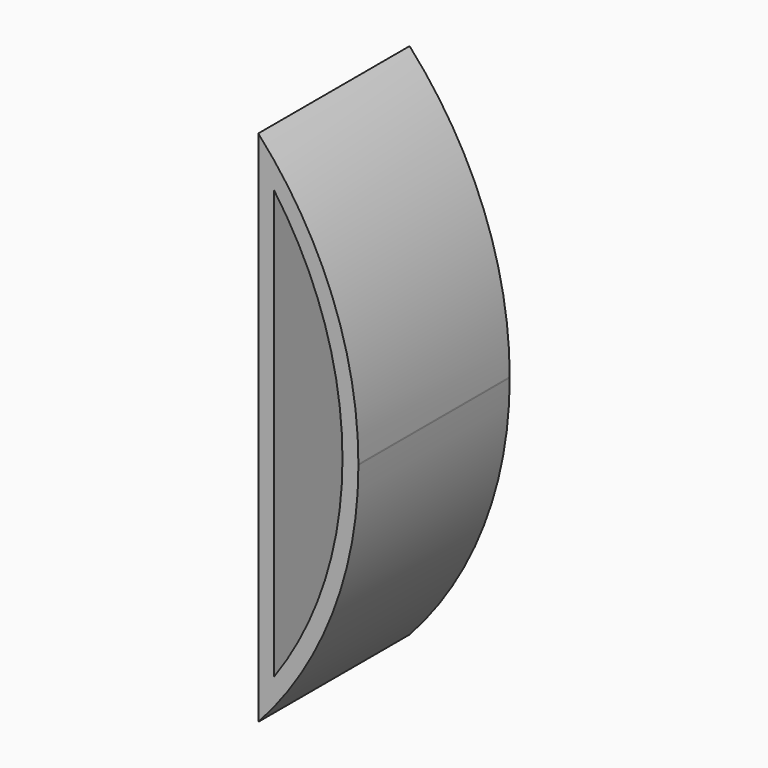
from build123d import *

# Parameters (mm, degrees)
F0_W        = 15.9461647272
F0_H        = 30.12368083
F1_DEPTH    = 82.5116038322
F2_T1_DEPTH = 236.0281493159
F3_T        = -2.54


# Not quite as in the source:
# - a fillet or chamfer that OpenCascade refuses, or shapes differently, is made with other operations: its cross-section is extruded or revolved along the edge and cut away or added


with BuildPart() as f1:
    # F0 (on Top) → F1 (new body)
    with BuildSketch(Plane.XY):
        with Locations((7.9730823636, 33.8614284992)):
            Rectangle(F0_W, F0_H)
    extrude(amount=F1_DEPTH)

    # F2: fillet of radius 61.1478122974 on 2 edges, made by hand

    # F2_s2 → F2_t1 (cut)
    with BuildSketch(Plane.XZ.offset(-151.8755031572)):
        with BuildLine():
            ThreePointArc((15.9461647272, 41.3307101351), (11.8204394221, 63.4109398395), (0, 82.5116038322))
            Line((0, 82.5116038322), (0.9040329514, 83.3352217062))
            ThreePointArc((0.9040329514, 83.3352217062), (7.9730823636, 83.7345600782), (15.9461647272, 83.7345600782))
            Line((15.9461647272, 83.7345600782), (17.1691209732, 82.5116038322))
            Line((17.1691209732, 82.5116038322), (17.1691209732, 41.3307101351))
            Line((17.1691209732, 41.3307101351), (15.9461647272, 41.3307101351))
        make_face()
        with BuildLine():
            ThreePointArc((15.9461647272, 41.1808936972), (11.8204394221, 19.1006639927), (0, 0))
            Line((0, 0), (0.9040329514, -0.8236178739))
            ThreePointArc((0.9040329514, -0.8236178739), (7.9730823636, -1.2229562459), (15.9461647272, -1.2229562459))
            Line((15.9461647272, -1.2229562459), (17.1691209732, 0))
            Line((17.1691209732, 0), (17.1691209732, 41.1808936972))
            Line((17.1691209732, 41.1808936972), (15.9461647272, 41.1808936972))
        make_face()
    extrude(amount=F2_T1_DEPTH, mode=Mode.SUBTRACT)

    # F3
    f3_openings = [f1.faces().sort_by_distance(p)[0] for p in [
        (6.459613, 18.799588, 41.255802),
    ]]
    offset(amount=F3_T, openings=f3_openings)


solid = f1.part
